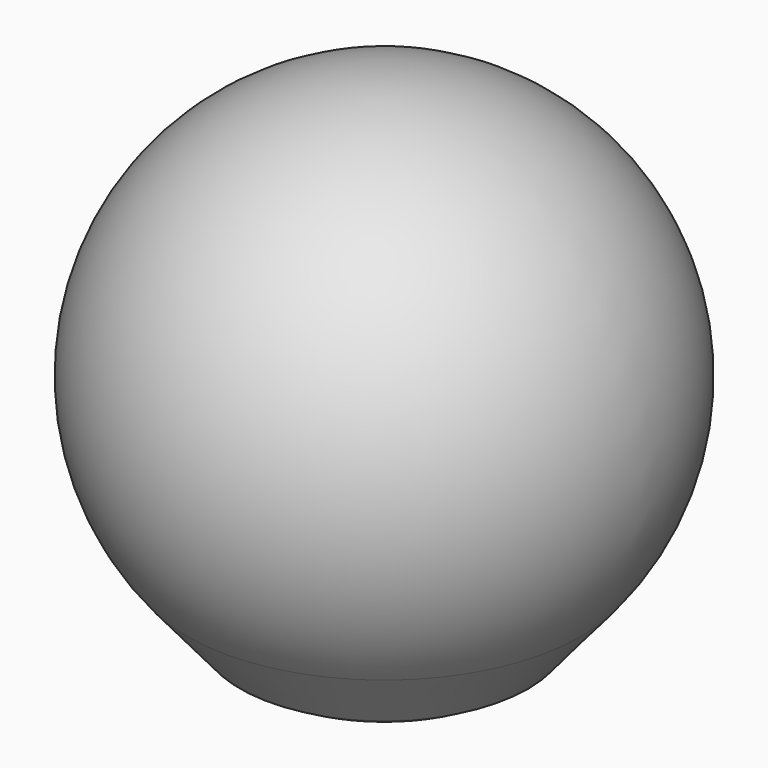
from build123d import *

# Parameters (mm, degrees)
F2_R     = 1.27
F3_DEPTH = 12.7
F4_SIZE  = 1.016
F7_R     = 2.286
F8_DEPTH = 25.4


# Not quite as in the source:
# - a feature names something its author has since deleted; it is built from what else it names


with BuildPart() as f1:
    # F0 (on Front) → F1 (revolve)
    with BuildSketch(Plane.XZ):
        with BuildLine():
            Line((16.7834315165, 0), (22.9813332936, 7.3863717094))
            ThreePointArc((22.9813332936, 7.3863717094), (27.1892336111, 39.3485478522), (0, 56.67))
            Line((0, 56.67), (0, 0))
            Line((0, 0), (16.7834315165, 0))
        make_face()
    revolve(axis=Axis((0, 0, -28.7515761617), (0, 0, -1)))

    # F2 (on face) → F3 (cut)
    with BuildSketch(Plane(origin=(0, 0, 0), x_dir=(1, 0, 0), z_dir=(0, 0, -1))):
        Circle(F2_R)
    extrude(amount=-F3_DEPTH, mode=Mode.SUBTRACT)

    # F4
    f4_edges = [f1.edges().sort_by_distance(p)[0] for p in [
        (-1.27, 0, 12.7),
    ]]
    chamfer(f4_edges, length=F4_SIZE)


with BuildPart() as f6:
    # F5 (on Front) → F6 (revolve)
    with BuildSketch(Plane.XZ):
        with BuildLine():
            Line((0, -1.016), (0, -4.8414657461))
            ThreePointArc((0, -4.8414657461), (8.7338903708, -3.6069158346), (16.7834315165, 0))
            Line((16.7834315165, 0), (10.4334315165, 0))
            Line((10.4334315165, 0), (10.4334315165, -1.016))
            Line((10.4334315165, -1.016), (0, -1.016))
        make_face()
    revolve(axis=Axis((0, 0, -28.7515761617), (0, 0, -1)))

    # F7 (on face) → F8 (cut)
    with BuildSketch(Plane.XY.offset(-1.016)):
        Circle(F7_R)
    extrude(amount=-F8_DEPTH, mode=Mode.SUBTRACT)


solid = Compound([f1.part, f6.part])
